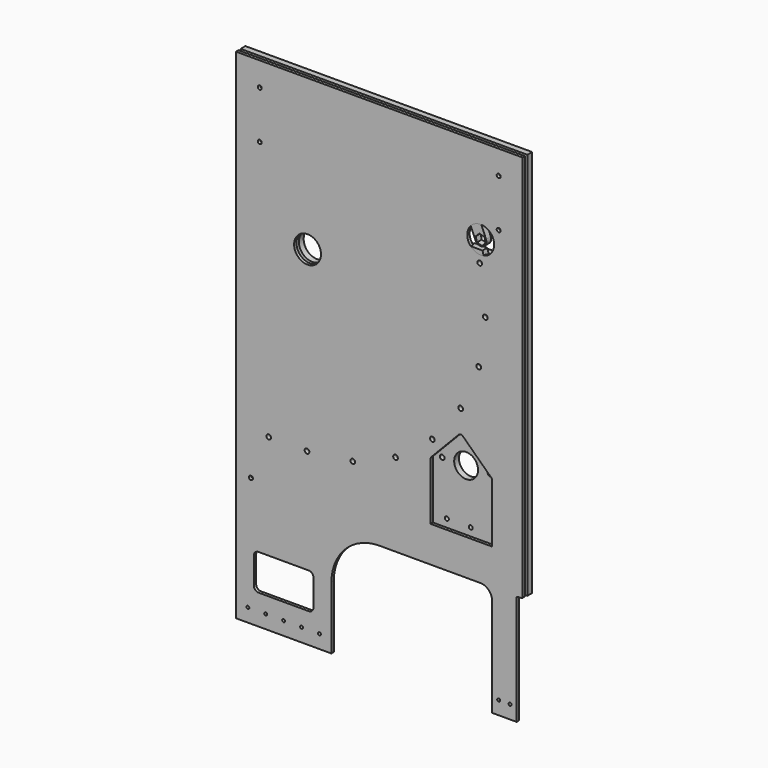
from build123d import *

# Parameters (mm, degrees)
F0_R      = 2.4892
F1_DEPTH  = 6.35
F2_R      = 2.1082
F2_R_2    = 2.4892
F2_R_3    = 12.7
F2_R_4    = 14.2875
F3_DEPTH  = 6.35
F4_R      = 2.4892
F4_W      = 63.5
F4_H      = 38.1
F4_R_2    = 2.1082
F4_R_3    = 14.2875
F4_W_2    = 65.5428959491
F4_W_3    = 25.9903480646
F4_H_2    = 92.075
F4_W_4    = 101.6
F4_H_3    = 22.225
F4_R_4    = 1.5875
F4_H_4    = 3.175
F4_W_5    = 6.35
F4_H_5    = 412.75
F5_DEPTH  = 3.175
F6_R      = 269.2084339335
F7_R      = 12.7
F8_R      = 5.08
F9_R      = 1.27
F11_DEPTH = 6.35
F12_R     = 12.7
F13_DEPTH = 12.7
F14_R     = 11.1125
F14_R_2   = 1.35255
F15_DEPTH = 6.35
F16_R     = 3.175


with BuildPart() as f1:
    # F0 (on Front) → F1 (new body)
    with BuildSketch(Plane.XZ):
        with BuildLine():
            ThreePointArc((172.6162349579, 59.4365361981), (148.6269643199, -106.014583352), (0, -182.5625))
            Line((0, -182.5625), (-41.275, -182.5625))
            Line((-41.275, -182.5625), (-76.2, -188.9125))
            Line((-76.2, -188.9125), (-76.2, -195.2625))
            Line((-76.2, -195.2625), (0, -195.2625))
            ThreePointArc((0, -195.2625), (157.6914242367, -115.1558015405), (185.9966184398, 59.4365361981))
            Line((185.9966184398, 59.4365361981), (172.6162349579, 59.4365361981))
        make_face()
        with Locations((-41.275, -188.9116044732)):
            Circle(F0_R, mode=Mode.SUBTRACT)
        with Locations((-0.5816799756, -188.9116044732)):
            Circle(F0_R, mode=Mode.SUBTRACT)
        with Locations((48.1043517168, -182.6852594003)):
            Circle(F0_R, mode=Mode.SUBTRACT)
        with Locations((93.5431218442, -164.12683209)):
            Circle(F0_R, mode=Mode.SUBTRACT)
        with Locations((132.667307669, -134.4891004212)):
            Circle(F0_R, mode=Mode.SUBTRACT)
        with Locations((162.8358494875, -95.772745486)):
            Circle(F0_R, mode=Mode.SUBTRACT)
        with Locations((182.0122341191, -50.5912965562)):
            Circle(F0_R, mode=Mode.SUBTRACT)
        with Locations((188.9019687672, -1.9947060235)):
            Circle(F0_R, mode=Mode.SUBTRACT)
        with Locations((183.0399651455, 46.7365361981)):
            Circle(F0_R, mode=Mode.SUBTRACT)
    extrude(amount=F1_DEPTH)

    # F6
    f6_edges = [f1.edges().sort_by_distance(p)[0] for p in [
        (-41.275, -3.175, -182.5625),
    ]]
    fillet(f6_edges, radius=F6_R)


with BuildPart() as f3:
    # F2 (on face) → F3 (new body)
    with BuildSketch(Plane.XZ):
        Polygon((-76.2, -195.2625), (-76.2, -252.4125), (228.6, -252.4125), (228.6, -195.2625), (0, -195.2625), align=None)
        with Locations((-60.198, -233.3625)):
            Circle(F2_R, mode=Mode.SUBTRACT)
        with Locations((-34.798, -233.3625)):
            Circle(F2_R, mode=Mode.SUBTRACT)
        with Locations((-60.198, -207.9625)):
            Circle(F2_R, mode=Mode.SUBTRACT)
        with Locations((-34.798, -207.9625)):
            Circle(F2_R, mode=Mode.SUBTRACT)
        with Locations((-9.398, -233.3625)):
            Circle(F2_R, mode=Mode.SUBTRACT)
        with Locations((16.002, -233.3625)):
            Circle(F2_R, mode=Mode.SUBTRACT)
        with Locations((-9.398, -207.9625)):
            Circle(F2_R, mode=Mode.SUBTRACT)
        with Locations((16.002, -207.9625)):
            Circle(F2_R, mode=Mode.SUBTRACT)
        with Locations((41.402, -233.3625)):
            Circle(F2_R, mode=Mode.SUBTRACT)
        with Locations((66.802, -233.3625)):
            Circle(F2_R, mode=Mode.SUBTRACT)
        with Locations((92.202, -233.3625)):
            Circle(F2_R, mode=Mode.SUBTRACT)
        with Locations((41.402, -207.9625)):
            Circle(F2_R, mode=Mode.SUBTRACT)
        with Locations((66.802, -207.9625)):
            Circle(F2_R, mode=Mode.SUBTRACT)
        with Locations((92.202, -207.9625)):
            Circle(F2_R, mode=Mode.SUBTRACT)
        with Locations((117.602, -233.3625)):
            Circle(F2_R, mode=Mode.SUBTRACT)
        with Locations((143.002, -233.3625)):
            Circle(F2_R, mode=Mode.SUBTRACT)
        with Locations((117.602, -207.9625)):
            Circle(F2_R, mode=Mode.SUBTRACT)
        with Locations((143.002, -207.9625)):
            Circle(F2_R, mode=Mode.SUBTRACT)
        with Locations((168.402, -233.3625)):
            Circle(F2_R, mode=Mode.SUBTRACT)
        with Locations((193.802, -233.3625)):
            Circle(F2_R, mode=Mode.SUBTRACT)
        with Locations((168.402, -207.9625)):
            Circle(F2_R, mode=Mode.SUBTRACT)
        with Locations((193.802, -207.9625)):
            Circle(F2_R, mode=Mode.SUBTRACT)
        with Locations((219.202, -233.3625)):
            Circle(F2_R, mode=Mode.SUBTRACT)
        with Locations((219.202, -207.9625)):
            Circle(F2_R, mode=Mode.SUBTRACT)
        with BuildLine():
            Line((0, -195.2625), (228.6, -195.2625))
            Line((228.6, -195.2625), (228.6, 160.3375))
            Line((228.6, 160.3375), (-76.2, 160.3375))
            Line((-76.2, 160.3375), (-76.2, -188.9125))
            Line((-76.2, -188.9125), (-41.275, -182.5625))
            Line((-41.275, -182.5625), (0, -182.5625))
            ThreePointArc((0, -182.5625), (148.6269643199, -106.014583352), (172.6162349579, 59.4365361981))
            Line((172.6162349579, 59.4365361981), (185.9966184398, 59.4365361981))
            ThreePointArc((185.9966184398, 59.4365361981), (157.6914242367, -115.1558015405), (0, -195.2625))
        make_face()
        with Locations((138.0932307091, -152.1824602719)):
            Circle(F2_R_2, mode=Mode.SUBTRACT)
        with Locations((163.4882039608, -151.6771548707)):
            Circle(F2_R_3, mode=Mode.SUBTRACT)
        with Locations((188.8831772124, -151.1718494695)):
            Circle(F2_R_2, mode=Mode.SUBTRACT)
        Circle(F2_R_4, mode=Mode.SUBTRACT)
        with Locations((-50.8, 84.1375)):
            Circle(F2_R, mode=Mode.SUBTRACT)
        with Locations((-50.8, 134.9375)):
            Circle(F2_R, mode=Mode.SUBTRACT)
        with Locations((203.2, 84.1375)):
            Circle(F2_R, mode=Mode.SUBTRACT)
        with Locations((203.2, 134.9375)):
            Circle(F2_R, mode=Mode.SUBTRACT)
        with BuildLine():
            Line((-76.2, -188.9125), (-76.2, -195.2625))
            Line((-76.2, -195.2625), (0, -195.2625))
            ThreePointArc((0, -195.2625), (157.6914242367, -115.1558015405), (185.9966184398, 59.4365361981))
            Line((185.9966184398, 59.4365361981), (172.6162349579, 59.4365361981))
            ThreePointArc((172.6162349579, 59.4365361981), (148.6269643199, -106.014583352), (0, -182.5625))
            Line((0, -182.5625), (-41.275, -182.5625))
            Line((-41.275, -182.5625), (-76.2, -188.9125))
        make_face()
        with Locations((-41.275, -188.9116044732)):
            Circle(F2_R_2, mode=Mode.SUBTRACT)
        with Locations((-0.5816799756, -188.9116044732)):
            Circle(F2_R_2, mode=Mode.SUBTRACT)
        with Locations((48.1043517168, -182.6852594003)):
            Circle(F2_R_2, mode=Mode.SUBTRACT)
        with Locations((93.5431218442, -164.12683209)):
            Circle(F2_R_2, mode=Mode.SUBTRACT)
        with Locations((132.667307669, -134.4891004212)):
            Circle(F2_R_2, mode=Mode.SUBTRACT)
        with Locations((162.8358494875, -95.772745486)):
            Circle(F2_R_2, mode=Mode.SUBTRACT)
        with Locations((182.0122341191, -50.5912965562)):
            Circle(F2_R_2, mode=Mode.SUBTRACT)
        with Locations((188.9019687672, -1.9947060235)):
            Circle(F2_R_2, mode=Mode.SUBTRACT)
        with Locations((183.0399651455, 46.7365361981)):
            Circle(F2_R_2, mode=Mode.SUBTRACT)
    extrude(amount=-F3_DEPTH)


with BuildPart() as f5:
    # F4 (on face) → F5 (new body)
    with BuildSketch(Plane.XZ.offset(6.35)):
        with BuildLine():
            Line((-41.275, -182.5625), (-76.2, -188.9125))
            Line((-76.2, -188.9125), (-76.2, -195.2625))
            Line((-76.2, -195.2625), (0, -195.2625))
            ThreePointArc((0, -195.2625), (157.6914242367, -115.1558015405), (185.9966184398, 59.4365361981))
            Line((185.9966184398, 59.4365361981), (172.6162349579, 59.4365361981))
            ThreePointArc((172.6162349579, 59.4365361981), (148.6269643199, -106.014583352), (0, -182.5625))
            Line((0, -182.5625), (-41.275, -182.5625))
        make_face()
        with Locations((-41.275, -188.9116044732)):
            Circle(F4_R, mode=Mode.SUBTRACT)
        with Locations((-0.5816799756, -188.9116044732)):
            Circle(F4_R, mode=Mode.SUBTRACT)
        with Locations((48.1043517168, -182.6852594003)):
            Circle(F4_R, mode=Mode.SUBTRACT)
        with Locations((93.5431218442, -164.12683209)):
            Circle(F4_R, mode=Mode.SUBTRACT)
        with Locations((132.667307669, -134.4891004212)):
            Circle(F4_R, mode=Mode.SUBTRACT)
        with Locations((162.8358494875, -95.772745486)):
            Circle(F4_R, mode=Mode.SUBTRACT)
        with Locations((182.0122341191, -50.5912965562)):
            Circle(F4_R, mode=Mode.SUBTRACT)
        with Locations((188.9019687672, -1.9947060235)):
            Circle(F4_R, mode=Mode.SUBTRACT)
        with Locations((183.0399651455, 46.7365361981)):
            Circle(F4_R, mode=Mode.SUBTRACT)
        with BuildLine():
            Line((222.25, 160.3375), (-76.2, 160.3375))
            Line((-76.2, 160.3375), (-76.2, -188.9125))
            Line((-76.2, -188.9125), (-41.275, -182.5625))
            Line((-41.275, -182.5625), (0, -182.5625))
            ThreePointArc((0, -182.5625), (148.6269643199, -106.014583352), (172.6162349579, 59.4365361981))
            Line((172.6162349579, 59.4365361981), (185.9966184398, 59.4365361981))
            ThreePointArc((185.9966184398, 59.4365361981), (157.6914242367, -115.1558015405), (0, -195.2625))
            Line((0, -195.2625), (-76.2, -195.2625))
            Line((-76.2, -195.2625), (-76.2, -252.4125))
            Line((-76.2, -252.4125), (-76.2, -344.4875))
            Line((-76.2, -344.4875), (25.4, -344.4875))
            Line((25.4, -344.4875), (25.4, -303.2125))
            ThreePointArc((25.4, -303.2125), (40.2789755157, -267.2914755157), (76.2, -252.4125))
            Line((76.2, -252.4125), (130.7167559862, -252.4125))
            Line((130.7167559862, -252.4125), (130.7167559862, -214.3125))
            Line((130.7167559862, -214.3125), (130.7167559862, -153.6075123877))
            ThreePointArc((130.7167559862, -153.6075123877), (130.7655648891, -153.0529366719), (130.9104909308, -152.5154118112))
            ThreePointArc((130.9104909308, -152.5154118112), (131.1988941232, -151.9255135807), (131.6024731525, -151.4075557729))
            Line((131.6024731525, -151.4075557729), (160.6361659477, -121.1949897299))
            ThreePointArc((160.6361659477, -121.1949897299), (162.8622856063, -120.2205746883), (165.1254053963, -121.105663511))
            Line((165.1254053963, -121.105663511), (195.2846085502, -150.0880755999))
            ThreePointArc((195.2846085502, -150.0880755999), (195.731151076, -150.6233153045), (196.0501334868, -151.24309913))
            ThreePointArc((196.0501334868, -151.24309913), (196.206832978, -151.8006344641), (196.2596519354, -152.3773584336))
            Line((196.2596519354, -152.3773584336), (196.2596519354, -214.3125))
            Line((196.2596519354, -214.3125), (196.2596519354, -252.4125))
            Line((196.2596519354, -252.4125), (222.25, -252.4125))
            Line((222.25, -252.4125), (222.25, 160.3375))
        make_face()
        with Locations((-25.4, -319.0875)):
            Rectangle(F4_W, F4_H, mode=Mode.SUBTRACT)
        with Locations((-60.198, -233.3625)):
            Circle(F4_R_2, mode=Mode.SUBTRACT)
        Circle(F4_R_3, mode=Mode.SUBTRACT)
        with Locations((-50.8, 84.1375)):
            Circle(F4_R_2, mode=Mode.SUBTRACT)
        with Locations((-50.8, 134.9375)):
            Circle(F4_R_2, mode=Mode.SUBTRACT)
        with Locations((203.2, 84.1375)):
            Circle(F4_R_2, mode=Mode.SUBTRACT)
        with Locations((203.2, 134.9375)):
            Circle(F4_R_2, mode=Mode.SUBTRACT)
        with Locations((163.4882039608, -233.3625)):
            Rectangle(F4_W_2, F4_H)
        with Locations((209.2548259677, -298.45)):
            Rectangle(F4_W_3, F4_H_2)
        with Locations((-25.4, -355.6)):
            Rectangle(F4_W_4, F4_H_3)
        with Locations((-63.5, -355.6)):
            Circle(F4_R_4, mode=Mode.SUBTRACT)
        with Locations((-44.45, -355.6)):
            Circle(F4_R_4, mode=Mode.SUBTRACT)
        with Locations((-25.4, -355.6)):
            Circle(F4_R_4, mode=Mode.SUBTRACT)
        with Locations((-6.35, -355.6)):
            Circle(F4_R_4, mode=Mode.SUBTRACT)
        with Locations((12.7, -355.6)):
            Circle(F4_R_4, mode=Mode.SUBTRACT)
        with Locations((209.2548259677, -355.6)):
            Rectangle(F4_W_3, F4_H_3)
        with Locations((203.2, -355.6)):
            Circle(F4_R_4, mode=Mode.SUBTRACT)
        with Locations((215.3096519354, -355.6)):
            Circle(F4_R_4, mode=Mode.SUBTRACT)
        with Locations((209.2548259677, -368.3)):
            Rectangle(F4_W_3, F4_H_4)
        with Locations((-25.4, -368.3)):
            Rectangle(F4_W_4, F4_H_4)
        with Locations((225.425, -46.0375)):
            Rectangle(F4_W_5, F4_H_5)
    extrude(amount=-F5_DEPTH)

    # F7
    f7_edges = [f5.edges().sort_by_distance(p)[0] for p in [
        (196.259652, -4.7625, -252.4125),
    ]]
    fillet(f7_edges, radius=F7_R)

    # F8
    f8_edges = [f5.edges().sort_by_distance(p)[0] for p in [
        (6.35, -4.7625, -300.0375),
        (-57.15, -4.7625, -300.0375),
        (-57.15, -4.7625, -338.1375),
        (6.35, -4.7625, -338.1375),
    ]]
    fillet(f8_edges, radius=F8_R)

    # F9
    f9_edges = [f5.edges().sort_by_distance(p)[0] for p in [
        (228.6, -4.7625, -252.4125),
        (222.25, -4.7625, -252.4125),
    ]]
    fillet(f9_edges, radius=F9_R)


with BuildPart() as f11:
    # F10 (on face) → F11 (new body)
    with BuildSketch(Plane.XZ.offset(6.35)):
        with BuildLine():
            ThreePointArc((173.5222104125, 78.6148363451), (176.0543788965, 72.7674767418), (178.3895682335, 66.8387009557))
            ThreePointArc((178.3895682335, 66.8387009557), (186.1781578503, 63.2957818237), (189.7210769822, 71.0843714404))
            ThreePointArc((189.7210769822, 71.0843714404), (187.3159849558, 77.1997195229), (184.7138345646, 83.2338526973))
            ThreePointArc((184.7138345646, 83.2338526973), (178.604564818, 82.168424392), (173.5222104125, 78.6148363451))
        make_face()
        Polygon((180.0979695106, 65.1429983283), (178.7696952587, 70.4794355772), (182.727048356, 74.297973447), (188.0126757052, 72.7800740679), (189.3409499571, 67.4436368189), (185.3835968598, 63.6250989492), align=None, mode=Mode.SUBTRACT)
        with BuildLine():
            ThreePointArc((138.9176072075, 130.3539351448), (158.3473823426, 105.9073014728), (173.5222104125, 78.6148363451))
            ThreePointArc((173.5222104125, 78.6148363451), (178.604564818, 82.168424392), (184.7138345646, 83.2338526973))
            ThreePointArc((184.7138345646, 83.2338526973), (171.5308794755, 107.8157330854), (155.0965070743, 130.3539351448))
            Line((155.0965070743, 130.3539351448), (138.9176072075, 130.3539351448))
        make_face()
    extrude(amount=-F11_DEPTH)

    # F12
    f12_edges = [f11.edges().sort_by_distance(p)[0] for p in [
        (155.096507, -3.175, 130.353935),
    ]]
    fillet(f12_edges, radius=F12_R)

    # F16
    f16_edges = [f11.edges().sort_by_distance(p)[0] for p in [
        (138.917607, -3.175, 130.353935),
    ]]
    fillet(f16_edges, radius=F16_R)


with BuildPart() as f13_tool:
    # F10 (on face) → F13 (new body, through all)
    with BuildSketch(Plane.XZ.offset(6.35)):
        with BuildLine():
            ThreePointArc((189.7210769822, 71.0843714404), (191.926580462, 64.8942418598), (193.9301751825, 58.6358428615))
            ThreePointArc((193.9301751825, 58.6358428615), (197.1934277302, 63.3470148431), (198.3428226079, 68.9615361981))
            ThreePointArc((198.3428226079, 68.9615361981), (194.388307313, 78.8287588739), (184.7138345646, 83.2338526973))
            ThreePointArc((184.7138345646, 83.2338526973), (187.3159849558, 77.1997195229), (189.7210769822, 71.0843714404))
        make_face()
        with BuildLine():
            ThreePointArc((173.5222104125, 78.6148363451), (170.6761049904, 63.9486336264), (182.4587818372, 54.7635182442))
            ThreePointArc((182.4587818372, 54.7635182442), (180.5251656877, 60.8351424214), (178.3895682335, 66.8387009557))
            ThreePointArc((178.3895682335, 66.8387009557), (176.0543788965, 72.7674767418), (173.5222104125, 78.6148363451))
        make_face()
        with BuildLine():
            ThreePointArc((173.5222104125, 78.6148363451), (176.0543788965, 72.7674767418), (178.3895682335, 66.8387009557))
            ThreePointArc((178.3895682335, 66.8387009557), (186.1781578503, 63.2957818237), (189.7210769822, 71.0843714404))
            ThreePointArc((189.7210769822, 71.0843714404), (187.3159849558, 77.1997195229), (184.7138345646, 83.2338526973))
            ThreePointArc((184.7138345646, 83.2338526973), (178.604564818, 82.168424392), (173.5222104125, 78.6148363451))
        make_face()
        Polygon((180.0979695106, 65.1429983283), (178.7696952587, 70.4794355772), (182.727048356, 74.297973447), (188.0126757052, 72.7800740679), (189.3409499571, 67.4436368189), (185.3835968598, 63.6250989492), align=None, mode=Mode.SUBTRACT)
        with BuildLine():
            ThreePointArc((178.3895682335, 66.8387009557), (180.5251656877, 60.8351424214), (182.4587818372, 54.7635182442))
            ThreePointArc((182.4587818372, 54.7635182442), (188.6249326641, 55.4245010654), (193.9301751825, 58.6358428615))
            ThreePointArc((193.9301751825, 58.6358428615), (191.926580462, 64.8942418598), (189.7210769822, 71.0843714404))
            ThreePointArc((189.7210769822, 71.0843714404), (186.1781578503, 63.2957818237), (178.3895682335, 66.8387009557))
        make_face()
        Polygon((182.727048356, 74.297973447), (178.7696952587, 70.4794355772), (180.0979695106, 65.1429983283), (185.3835968598, 63.6250989492), (189.3409499571, 67.4436368189), (188.0126757052, 72.7800740679), align=None)
    extrude(amount=-F13_DEPTH)


with BuildPart() as f3_1:
    add(f3.part)

    # F13: cut by f13_tool
    add(f13_tool.part, mode=Mode.SUBTRACT)

    # F14 (on face) → F15 (cut, through all)
    with BuildSketch(Plane(origin=(0, 6.35, 0), x_dir=(-1, 0, 0), z_dir=(0, 1, 0))):
        with BuildLine():
            ThreePointArc((-138.5276006076, 78.6075042328), (-136.8460695578, 81.3500616095), (-139.2921406076, 83.4395361978))
            Line((-139.2921406076, 83.4395361978), (-197.4530606076, 83.4395361978))
            ThreePointArc((-197.4530606076, 83.4395361978), (-199.8991316575, 81.3500616095), (-198.2176006076, 78.6075042328))
            Line((-198.2176006076, 78.6075042328), (-198.2176006076, 71.4380361978))
            Line((-198.2176006076, 71.4380361978), (-202.3451006074, 71.4380361978))
            ThreePointArc((-202.3451006074, 71.4380361978), (-204.8216006074, 68.9615361978), (-202.3451006074, 66.4850361978))
            Line((-202.3451006074, 66.4850361978), (-198.2176006084, 66.4850361978))
            Line((-198.2176006084, 66.4850361978), (-198.2176006084, 59.3155681631))
            ThreePointArc((-198.2176006084, 59.3155681631), (-199.8991316579, 56.5730107864), (-197.4530606081, 54.4835361982))
            Line((-197.4530606081, 54.4835361982), (-139.2921406081, 54.4835361982))
            ThreePointArc((-139.2921406081, 54.4835361982), (-136.8460695583, 56.5730107864), (-138.5276006079, 59.3155681631))
            Line((-138.5276006079, 59.3155681631), (-138.5276006079, 66.4850361978))
            Line((-138.5276006079, 66.4850361978), (-134.4001006079, 66.4850361978))
            ThreePointArc((-134.4001006079, 66.4850361978), (-131.9236006079, 68.9615361978), (-134.4001006079, 71.4380361978))
            Line((-134.4001006079, 71.4380361978), (-138.5276006076, 71.4380361978))
            Line((-138.5276006076, 71.4380361978), (-138.5276006076, 78.6075042328))
        make_face()
        with Locations((-184.0553226079, 68.9615361981)):
            Circle(F14_R, mode=Mode.SUBTRACT)
        with Locations((-202.0276006079, 61.0875361981)):
            Circle(F14_R_2)
        with Locations((-202.0276006079, 76.8355361981)):
            Circle(F14_R_2)
        with Locations((-134.7176006079, 61.0875361981)):
            Circle(F14_R_2)
        with Locations((-134.7176006079, 76.8355361981)):
            Circle(F14_R_2)
        with Locations((-184.0553226079, 68.9615361981)):
            Circle(F14_R)
    extrude(amount=-F15_DEPTH, mode=Mode.SUBTRACT)


with BuildPart() as f5_1:
    add(f5.part)

    # F13: cut by f13_tool
    add(f13_tool.part, mode=Mode.SUBTRACT)


solid = Compound([f1.part, f11.part, f3_1.part, f5_1.part])
